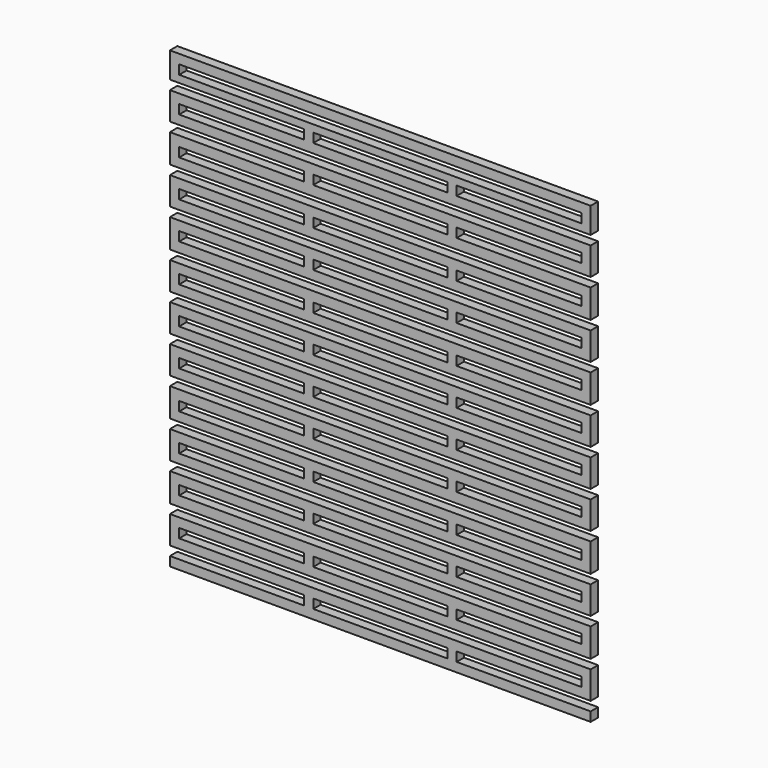
from build123d import *

# Parameters (mm, degrees)
F0_W     = 87
F0_H     = 2
F0_W_2   = 29
F1_DEPTH = 2


# Not quite as in the source:
# - ends of sketch curves that miss each other by under 0.0002 mm in the source are joined


with BuildPart() as f1:
    # F0 (on Front) → F1 (new body)
    with BuildSketch(Plane.XZ):
        Polygon((-74.1755201817, -53.7046223087), (-74.1755201817, -54.8843706005), (16.8244798183, -54.8843706005), (16.8244798183, -52.8843706005), (-12.1755201817, -52.8843706005), (-12.1755201817, -50.8843706005), (16.8244798183, -50.8843706005), (16.8244798183, -44.8844749875), (-12.1755201817, -44.8844749875), (-12.1755201817, -42.8844749875), (16.8244798183, -42.8844749875), (16.8244798183, -36.7078750432), (-12.1755201817, -36.7078750432), (-12.1754285991, -34.7078750432), (16.8244798183, -34.7078750432), (16.8244798183, -28.7078750432), (-12.1755201817, -28.7078750432), (-12.1754285991, -26.7078750432), (16.8244798183, -26.7078750432), (16.8244798183, -20.5312750988), (-12.1755201817, -20.5312750988), (-12.1755201817, -18.5312750988), (16.8244798183, -18.5312750988), (16.8244798183, -12.5313794858), (-12.1755201817, -12.5313794858), (-12.1755201817, -10.5313794858), (16.8244798183, -10.5313794858), (16.8244798183, -4.5313794858), (-12.1755201817, -4.5313794858), (-12.1755201817, -2.5313794858), (16.8244798183, -2.5313794858), (16.8244798183, 3.4685161272), (-12.1755201817, 3.4685161272), (-12.1755201817, 5.4685161272), (16.8244798183, 5.4685161272), (16.8244798183, 11.6451160715), (-12.1755201817, 11.6451160715), (-12.1754285991, 13.6451160715), (16.8244798183, 13.6451160715), (16.8244798183, 19.6451160715), (-12.1755201817, 19.6451160715), (-12.1754285991, 21.6451160715), (16.8244798183, 21.6451160715), (16.8244798183, 27.8217160159), (-12.1755201817, 27.8217160159), (-12.1755201817, 29.8217160159), (16.8244798183, 29.8217160159), (16.8244798183, 35.8216116289), (-12.1755201817, 35.8216116289), (-12.1755201817, 37.8216116289), (16.8244798183, 37.8216116289), (16.8244798183, 43.3868200481), (-74.1755201817, 43.3868200481), (-74.1755201817, 37.8216116289), (-45.1755201817, 37.8216116289), (-45.1755201817, 35.8216116289), (-74.1755201817, 35.8216116289), (-74.1755201817, 29.8217160159), (-45.1755201817, 29.8217160159), (-45.1755201817, 27.8217160159), (-74.1755201817, 27.8217160159), (-74.1755201817, 21.6451160715), (-45.1755201817, 21.6451160715), (-45.1754285991, 19.6451160715), (-74.1755201817, 19.6451160715), (-74.1755201817, 13.6451160715), (-45.1755201817, 13.6451160715), (-45.1754285991, 11.6451160715), (-74.1755201817, 11.6451160715), (-74.1755201817, 5.4685161272), (-45.1755201817, 5.4685161272), (-45.1755201817, 3.4685161272), (-74.1755201817, 3.4685161272), (-74.1755201817, -2.5313794858), (-45.1755201817, -2.5313794858), (-45.1755201817, -4.5313794858), (-74.1755201817, -4.5313794858), (-74.1755201817, -10.5313794858), (-45.1755201817, -10.5313794858), (-45.1755201817, -12.5313794858), (-74.1755201817, -12.5313794858), (-74.1755201817, -18.5312750988), (-45.1755201817, -18.5312750988), (-45.1755201817, -20.5312750988), (-74.1755201817, -20.5312750988), (-74.1755201817, -26.7078750432), (-45.1755201817, -26.7078750432), (-45.1754285991, -28.7078750432), (-74.1755201817, -28.7078750432), (-74.1755201817, -34.7078750432), (-45.1755201817, -34.7078750432), (-45.1754285991, -36.7078750432), (-74.1755201817, -36.7078750432), (-74.1755201817, -42.8844749875), (-45.1755201817, -42.8844749875), (-45.1755201817, -44.8844749875), (-74.1755201817, -44.8844749875), (-74.1755201817, -50.8843706005), (-45.1755201817, -50.8843706005), (-45.1755201817, -52.8843706005), (-74.1755201817, -52.8843706005), align=None)
        with Locations((-28.6755201817, -47.8843706005)):
            Rectangle(F0_W, F0_H, mode=Mode.SUBTRACT)
        with Locations((-28.6755201817, -43.8844749875)):
            Rectangle(F0_W_2, F0_H, mode=Mode.SUBTRACT)
        with Locations((-28.6755201817, -31.7078686953)):
            Rectangle(F0_W, F0_H, mode=Mode.SUBTRACT)
        with Locations((-28.6755201817, -19.5312750988)):
            Rectangle(F0_W_2, F0_H, mode=Mode.SUBTRACT)
        with Locations((-28.6755201817, -15.5313794858)):
            Rectangle(F0_W, F0_H, mode=Mode.SUBTRACT)
        with Locations((-28.6755201817, -51.8843706005)):
            Rectangle(F0_W_2, F0_H, mode=Mode.SUBTRACT)
        with Locations((-28.6754285991, -39.7078750432)):
            Rectangle(F0_W, F0_H, mode=Mode.SUBTRACT)
        with Locations((-28.6754285991, -35.7078750432)):
            Rectangle(F0_W_2, F0_H, mode=Mode.SUBTRACT)
        with Locations((-28.6754285991, -27.7078750432)):
            Rectangle(F0_W_2, F0_H, mode=Mode.SUBTRACT)
        with Locations((-28.6754285991, -23.7078750432)):
            Rectangle(F0_W, F0_H, mode=Mode.SUBTRACT)
        with Locations((-28.6755201817, -11.5313794858)):
            Rectangle(F0_W_2, F0_H, mode=Mode.SUBTRACT)
        with Locations((-28.6755201817, -7.5313794858)):
            Rectangle(F0_W, F0_H, mode=Mode.SUBTRACT)
        with Locations((-28.6755201817, 0.4686205142)):
            Rectangle(F0_W, F0_H, mode=Mode.SUBTRACT)
        with Locations((-28.6755201817, 4.4685161272)):
            Rectangle(F0_W_2, F0_H, mode=Mode.SUBTRACT)
        with Locations((-28.6755201817, 16.6451224194)):
            Rectangle(F0_W, F0_H, mode=Mode.SUBTRACT)
        with Locations((-28.6755201817, 28.8217160159)):
            Rectangle(F0_W_2, F0_H, mode=Mode.SUBTRACT)
        with Locations((-28.6755201817, 32.8216116289)):
            Rectangle(F0_W, F0_H, mode=Mode.SUBTRACT)
        with Locations((-28.6755201817, 40.3868200481)):
            Rectangle(F0_W, F0_H, mode=Mode.SUBTRACT)
        with Locations((-28.6755201817, -3.5313794858)):
            Rectangle(F0_W_2, F0_H, mode=Mode.SUBTRACT)
        with Locations((-28.6754285991, 8.6451160715)):
            Rectangle(F0_W, F0_H, mode=Mode.SUBTRACT)
        with Locations((-28.6754285991, 12.6451160715)):
            Rectangle(F0_W_2, F0_H, mode=Mode.SUBTRACT)
        with Locations((-28.6754285991, 20.6451160715)):
            Rectangle(F0_W_2, F0_H, mode=Mode.SUBTRACT)
        with Locations((-28.6754285991, 24.6451160715)):
            Rectangle(F0_W, F0_H, mode=Mode.SUBTRACT)
        with Locations((-28.6755201817, 36.8216116289)):
            Rectangle(F0_W_2, F0_H, mode=Mode.SUBTRACT)
    extrude(amount=F1_DEPTH)


solid = f1.part
